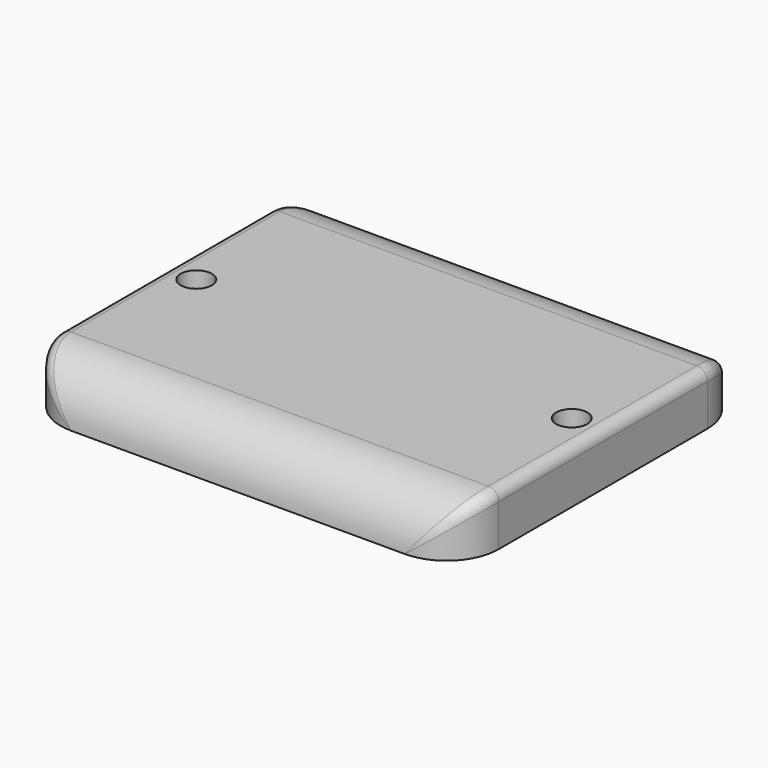
from build123d import *

# Parameters (mm, degrees)
F0_W     = 42
F0_H     = 35
F1_DEPTH = 5
F2_R     = 4.99999
F3_R     = 1.5
F4_DEPTH = 6
F5_F1_R  = 1
F5_F2_R  = 1


# Not quite as in the source:
# - a fillet or chamfer is up to 0.001 mm smaller than in the source, because OpenCascade refuses the exact size


with BuildPart() as f1:
    # F0 (on Top) → F1 (new body)
    with BuildSketch(Plane.XY):
        Rectangle(F0_W, F0_H)
    extrude(amount=F1_DEPTH)

    # F2 (radius 5 in the source; OpenCascade refuses exactly that, so slightly less here)
    f2_edges = [f1.edges().sort_by_distance(p)[0] for p in [
        (-21, -17.5, 2.5),
        (21, -17.5, 2.5),
        (-21, 17.5, 2.5),
        (21, 17.5, 2.5),
        (0, 17.5, 5),
        (0, -17.5, 5),
    ]]
    fillet(f2_edges, radius=F2_R)

    # F3 (on face) → F4 (cut)
    with BuildSketch(Plane.XY.offset(5)):
        with Locations((-18, 0)):
            Circle(F3_R)
        with Locations((18, 0)):
            Circle(F3_R)
    extrude(amount=-F4_DEPTH, mode=Mode.SUBTRACT)

    # F5: fillet of radius 1 on 2 edges, made by hand

    # F5_f1
    f5_f1_edges = [f1.edges().sort_by_distance(p)[0] for p in [
        (19.5355368349, 16.0355368349, 3.5355368349),
        (21, 0, 5),
        (19.5355368349, -16.0355368349, 3.5355368349),
    ]]
    fillet(f5_f1_edges, radius=F5_F1_R)

    # F5_f2
    f5_f2_edges = [f1.edges().sort_by_distance(p)[0] for p in [
        (-19.5355368349, 16.0355368349, 3.5355368349),
        (-21, 0, 5),
        (-19.5355368349, -16.0355368349, 3.5355368349),
    ]]
    fillet(f5_f2_edges, radius=F5_F2_R)


solid = f1.part
